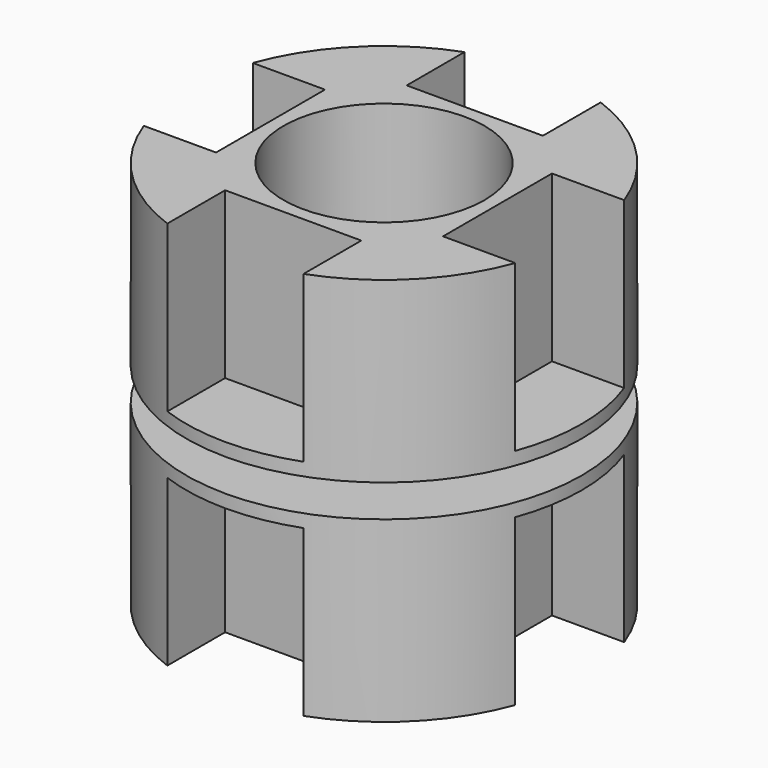
from build123d import *

# Parameters (mm, degrees)
F4_W            = 21
F4_H            = 25.5
F6_DEPTH        = 13.001
F6_COPIES_COUNT = 4


# Not quite as in the source:
# - a pattern or mirror of a feature is missing from the dataset's text; its kind, count and spacing are read off the source's solid


with BuildPart() as f5:
    # F2 (on Front) → F5 (revolve)
    with BuildSketch(Plane.XZ):
        Polygon((15.5, 30), (15.5, 0), (17.5, 0), (17.5, 2.5), (30.5, 2.5), (30.5, 30), align=None)
    revolve(axis=Axis((0, 0, 6.4842129506), (0, 0, -1)))

    # F4 (on offset) → F6 (cut, through all)
    with BuildSketch(Plane.YZ.offset(17.5)):
        with Locations((0, 17.25)):
            Rectangle(F4_W, F4_H)
    f6 = extrude(amount=F6_DEPTH, mode=Mode.SUBTRACT)

    # F6_copies: F6 ×4 about axis
    f6_copies_axis = Axis((0, 0, 0), (0, 0, 1))
    for i in range(1, F6_COPIES_COUNT):
        add(f6.rotate(f6_copies_axis, i * 360 / F6_COPIES_COUNT), mode=Mode.SUBTRACT)

    # F7: F5 across plane


with BuildPart() as f5_1:
    add(f5.part)
    add(f5.part.mirror(Plane.XY))


solid = f5_1.part
